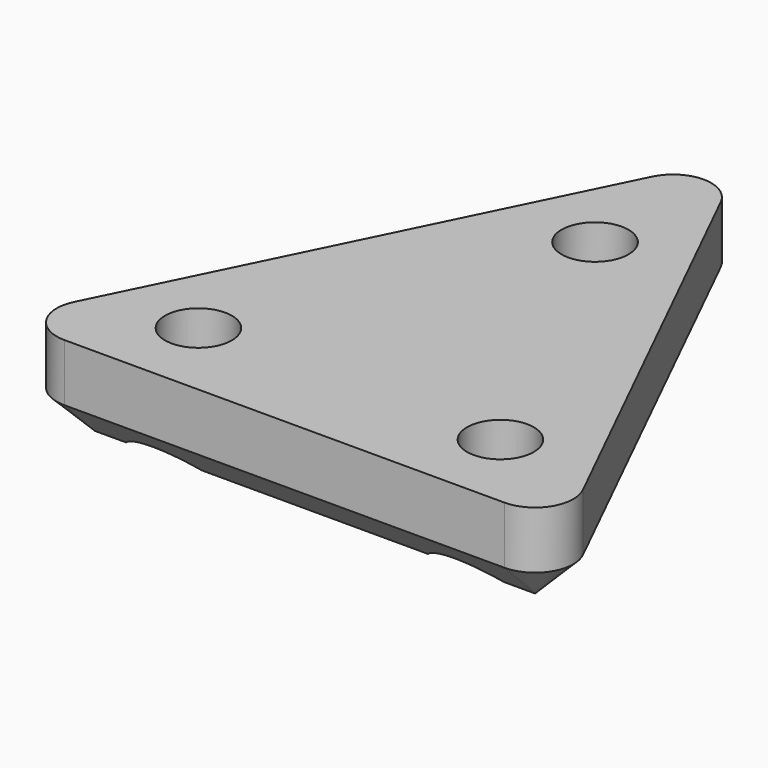
from build123d import *

# Parameters (mm, degrees)
F0_R         = 1.75
F1_DEPTH     = 5
F2_R         = 3
F3_DEPTH     = 3
F4_T1_DEPTH  = 23.0280702819
F4_T3_DEPTH  = 26.0887631675
F4_T5_DEPTH  = 26.0887631675
F4_T8_ANGLE  = 116.1894596418
F4_T10_ANGLE = 116.1894596418
F4_T12_ANGLE = 127.6210807165


# Not quite as in the source:
# - a fillet or chamfer that OpenCascade refuses, or shapes differently, is made with other operations: its cross-section is extruded or revolved along the edge and cut away or added


with BuildPart() as f1:
    # F0 (on Top) → F1 (new body)
    with BuildSketch(Plane.XY):
        with BuildLine():
            Line((6.1053208487, 22.0431612343), (-5.4087142923, -1.3673184358))
            ThreePointArc((-5.4087142923, -1.3673184358), (-5.3118812954, -3.3070328452), (-3.6140351409, -4.25))
            Line((-3.6140351409, -4.25), (19.4140351409, -4.25))
            ThreePointArc((19.4140351409, -4.25), (21.1118812954, -3.3070328452), (21.2087142923, -1.3673184358))
            Line((21.2087142923, -1.3673184358), (9.6946791513, 22.0431612343))
            ThreePointArc((9.6946791513, 22.0431612343), (7.9, 23.16047967), (6.1053208487, 22.0431612343))
        make_face()
        Circle(F0_R, mode=Mode.SUBTRACT)
        with Locations((15.8, 0)):
            Circle(F0_R, mode=Mode.SUBTRACT)
        with Locations((7.9, 16.0623784042)):
            Circle(F0_R, mode=Mode.SUBTRACT)
    extrude(amount=F1_DEPTH)

    # F2 (on Top) → F3 (cut)
    with BuildSketch(Plane.XY):
        with Locations((15.8, 0)):
            Circle(F2_R)
        Circle(F2_R)
        with Locations((7.9, 16.0623784042)):
            Circle(F2_R)
    extrude(amount=F3_DEPTH, mode=Mode.SUBTRACT)

    # F4: chamfer of 2 on 1 edges, made by hand

    # F4_s2 → F4_t1 (cut)
    with BuildSketch(Plane.YZ.offset(-3.6140351409)):
        Polygon((-2.25, 0), (-4.25, 2), (-4.25, 0), align=None)
    extrude(amount=F4_T1_DEPTH, mode=Mode.SUBTRACT)

    # F4_s4 → F4_t3 (cut)
    with BuildSketch(Plane(origin=(4.672571734, -9.5003310521, 0), x_dir=(0, 0, 1), z_dir=(-0.4413407821, 0.8973395757, 0))):
        Polygon((2, 18.4279652953), (0, 16.4279652953), (0, 18.4279652953), align=None)
    extrude(amount=F4_T3_DEPTH, mode=Mode.SUBTRACT)

    # F4_s6 → F4_t5 (cut)
    with BuildSketch(Plane(origin=(9.9190140452, 20.1674629103, 0), x_dir=(0, 0, 1), z_dir=(-0.4413407821, -0.8973395757, 0))):
        Polygon((2, 4.25), (0, 2.25), (0, 4.25), align=None)
    extrude(amount=F4_T5_DEPTH, mode=Mode.SUBTRACT)

    # F4_s7 → F4_t8 (revolve, cut)
    with BuildSketch(Plane(origin=(-1.5950210957, -3.2430167598, 0), x_dir=(0, 0, 1), z_dir=(0.4413407821, 0.8973395757, 0))):
        Polygon((0, -2.25), (2, -4.25), (0, -4.25), align=None)
    revolve(axis=Axis((-3.6140351409, -2.25, 0), (0, 0, 1)), revolution_arc=F4_T8_ANGLE, mode=Mode.SUBTRACT)

    # F4_s9 → F4_t10 (revolve, cut)
    with BuildSketch(Plane.YZ.offset(19.4140351409)):
        Polygon((-2.25, 0), (-4.25, 2), (-4.25, 0), align=None)
    revolve(axis=Axis((19.4140351409, -2.25, 0), (0, 0, 1)), revolution_arc=F4_T10_ANGLE, mode=Mode.SUBTRACT)

    # F4_s11 → F4_t12 (revolve, cut)
    with BuildSketch(Plane(origin=(-6.841463407, 13.9101486179, 0), x_dir=(0, 0, 1), z_dir=(0.4413407821, -0.8973395757, 0))):
        Polygon((2, -18.4279652953), (0, -16.4279652953), (0, -18.4279652953), align=None)
    revolve(axis=Axis((7.9, 21.16047967, 0), (0, 0, 1)), revolution_arc=F4_T12_ANGLE, mode=Mode.SUBTRACT)


solid = f1.part
